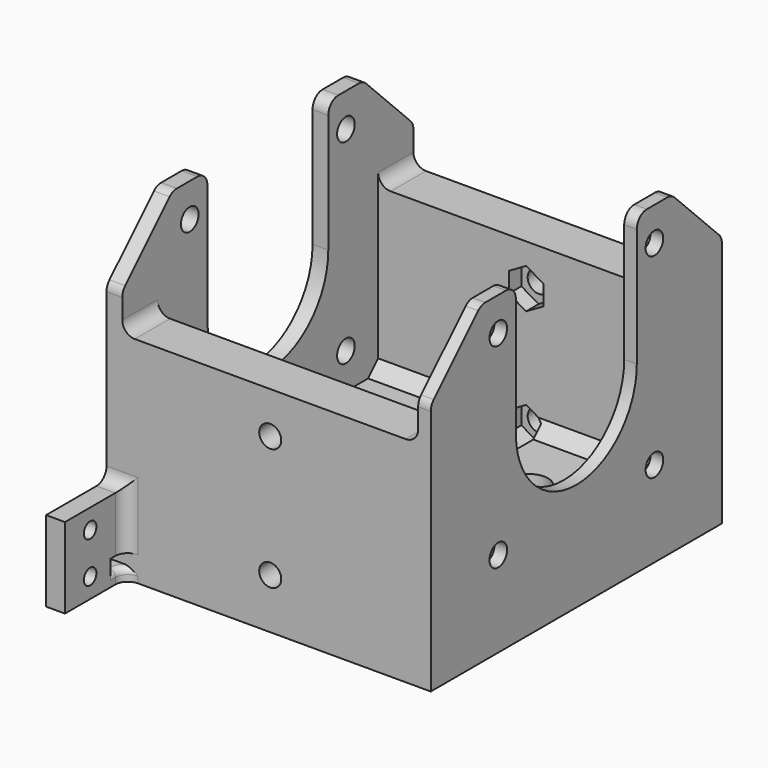
from build123d import *

# Parameters (mm, degrees)
F1_W         = 27
F1_H         = 43.8
F1_R         = 1.5
F1_H_2       = 7
F2_DEPTH     = 34
F3_R         = 1.75
F4_DEPTH     = 57.801
F5_W         = 43.8
F5_H         = 26
F6_DEPTH     = 27.001
F7_DEPTH     = 10
F8_DEPTH     = 10
F9_T4_DEPTH  = 26.8933659759
F9_S5_R      = 1.75
F9_T6_DEPTH  = 15
F9_T10_DEPTH = 26.8933659759
F9_S11_R     = 1.75
F9_T12_DEPTH = 15
F9_T16_DEPTH = 26.8933659759
F9_S17_R     = 1.75
F9_T18_DEPTH = 15
F9_T22_DEPTH = 26.8933659759
F9_S23_R     = 1.75
F9_T24_DEPTH = 15
F12_DEPTH    = 2.5
F14_DEPTH    = 2
F15_SIZE     = 10
F16_R        = 1.75
F17_DEPTH    = 51.5
F18_R        = 3
F19_DEPTH    = 4
F21_DEPTH    = 2.5
F22_DEPTH    = 47
F24_DEPTH    = 2.5
F25_R        = 1.25
F26_DEPTH    = 3
F27_R        = 2
F28_T1_DEPTH = 1
F28_T3_DEPTH = 3
F28_T8_ANGLE = 161.6484946187


# Not quite as in the source:
# - a fillet or chamfer that OpenCascade refuses, or shapes differently, is made with other operations: its cross-section is extruded or revolved along the edge and cut away or added


with BuildPart() as f2:
    # F1 (on Top) → F2 (new body)
    with BuildSketch(Plane.XY):
        Rectangle(F1_W, F1_H)
        with Locations((-10, -10)):
            Circle(F1_R, mode=Mode.SUBTRACT)
        with Locations((10, -10)):
            Circle(F1_R, mode=Mode.SUBTRACT)
        with Locations((-10, 10)):
            Circle(F1_R, mode=Mode.SUBTRACT)
        with Locations((10, 10)):
            Circle(F1_R, mode=Mode.SUBTRACT)
        with Locations((0, 25.4)):
            Rectangle(F1_W, F1_H_2)
        with Locations((0, -25.4)):
            Rectangle(F1_W, F1_H_2)
    extrude(amount=F2_DEPTH)

    # F3 (on face) → F4 (cut, through all)
    with BuildSketch(Plane(origin=(0, 28.9, 0), x_dir=(-1, 0, 0), z_dir=(0, 1, 0))):
        with Locations((0, 27.395)):
            Circle(F3_R)
        with Locations((0, 8)):
            Circle(F3_R)
    extrude(amount=-F4_DEPTH, mode=Mode.SUBTRACT)

    # F5 (on face) → F6 (cut, through all)
    with BuildSketch(Plane(origin=(-13.5, 0, 0), x_dir=(0, -1, 0), z_dir=(-1, 0, 0))):
        with Locations((0, 21)):
            Rectangle(F5_W, F5_H)
    extrude(amount=-F6_DEPTH, mode=Mode.SUBTRACT)

    # F7 (add): a face of the model
    f7_faces = [f2.faces().sort_by_distance(p)[0] for p in [
        (-13.5, 0, 0.6705848194),
    ]]
    extrude(f7_faces, amount=F7_DEPTH)

    # F8 (add): a face of the model
    f8_faces = [f2.faces().sort_by_distance(p)[0] for p in [
        (13.5, 0, 0.6705848194),
    ]]
    extrude(f8_faces, amount=F8_DEPTH)

    # F9: chamfer of 2 on 4 edges, made by hand


with BuildPart() as f9_tool2:
    # F9_s3 → F9_t4 (new body)
    with BuildSketch(Plane.YZ.offset(3.3933659759)):
        Polygon((-21.9, 10), (-19.9, 8), (-21.9, 8), align=None)
    extrude(amount=-F9_T4_DEPTH)

    # F9_s5 → F9_t6 (cut, symmetric)
    with BuildSketch(Plane.XZ.offset(20.9)):
        with Locations((0, 8)):
            Circle(F9_S5_R)
    extrude(amount=F9_T6_DEPTH, both=True, mode=Mode.SUBTRACT)


with BuildPart() as f2_1:
    add(f2.part)

    # F9_t1: union F9_tool2
    add(f9_tool2.part)


with BuildPart() as f9_tool8:
    # F9_s9 → F9_t10 (new body)
    with BuildSketch(Plane.YZ.offset(-23.5)):
        Polygon((21.9, 10), (19.9, 8), (21.9, 8), align=None)
    extrude(amount=F9_T10_DEPTH)

    # F9_s11 → F9_t12 (cut, symmetric)
    with BuildSketch(Plane.XZ.offset(-20.9)):
        with Locations((0, 8)):
            Circle(F9_S11_R)
    extrude(amount=F9_T12_DEPTH, both=True, mode=Mode.SUBTRACT)


with BuildPart() as f2_2:
    add(f2_1.part)

    # F9_t7: union F9_tool8
    add(f9_tool8.part)


with BuildPart() as f9_tool14:
    # F9_s15 → F9_t16 (new body)
    with BuildSketch(Plane.YZ.offset(-3.3933659759)):
        Polygon((21.9, 10), (19.9, 8), (21.9, 8), align=None)
    extrude(amount=F9_T16_DEPTH)

    # F9_s17 → F9_t18 (cut, symmetric)
    with BuildSketch(Plane.XZ.offset(-20.9)):
        with Locations((0, 8)):
            Circle(F9_S17_R)
    extrude(amount=F9_T18_DEPTH, both=True, mode=Mode.SUBTRACT)


with BuildPart() as f2_3:
    add(f2_2.part)

    # F9_t13: union F9_tool14
    add(f9_tool14.part)


with BuildPart() as f9_tool20:
    # F9_s21 → F9_t22 (new body)
    with BuildSketch(Plane.YZ.offset(23.5)):
        Polygon((-19.9, 8), (-21.9, 10), (-21.9, 8), align=None)
    extrude(amount=-F9_T22_DEPTH)

    # F9_s23 → F9_t24 (cut, symmetric)
    with BuildSketch(Plane.XZ.offset(20.9)):
        with Locations((0, 8)):
            Circle(F9_S23_R)
    extrude(amount=F9_T24_DEPTH, both=True, mode=Mode.SUBTRACT)


with BuildPart() as f2_4:
    add(f2_3.part)

    # F9_t19: union F9_tool20
    add(f9_tool20.part)

    # F11 (on face) → F12 (join)
    with BuildSketch(Plane(origin=(-23.5, 0, 0), x_dir=(0, -1, 0), z_dir=(-1, 0, 0))):
        Polygon((-28.9, 50), (-28.9, 34), (-28.9, 0), (28.9, 0), (28.9, 50), align=None)
    extrude(amount=F12_DEPTH)

    # F13 (on face) → F14 (join)
    with BuildSketch(Plane.YZ.offset(23.5)):
        Polygon((-28.9, 34), (-28.9, 28), (-28.9, 0), (28.9, 0), (28.9, 28), (28.9, 34), (28.9, 50), (-28.9, 50), align=None)
    extrude(amount=F14_DEPTH)

    # F15
    f15_edges = [f2_4.edges().sort_by_distance(p)[0] for p in [
        (-24.75, 28.9, 50),
        (-24.75, -28.9, 50),
        (24.5, -28.9, 50),
        (24.5, 28.9, 50),
    ]]
    chamfer(f15_edges, length=F15_SIZE)

    # F16 (on face) → F17 (cut, through all)
    with BuildSketch(Plane.YZ.offset(25.5)):
        with BuildLine():
            Line((-12, 50), (-12, 29.15))
            ThreePointArc((-12, 29.15), (0, 17.15), (12, 29.15))
            Line((12, 29.15), (12, 50))
            Line((12, 50), (-12, 50))
        make_face()
        with Locations((-15.5, 44.65)):
            Circle(F16_R)
        with Locations((15.5, 44.65)):
            Circle(F16_R)
        with Locations((15.5, 13.65)):
            Circle(F16_R)
        with Locations((-15.5, 13.65)):
            Circle(F16_R)
    extrude(amount=-F17_DEPTH, mode=Mode.SUBTRACT)

    # F18 (on face) → F19 (cut)
    with BuildSketch(Plane.XY.offset(8)):
        with Locations((10, -10)):
            Circle(F18_R)
        with Locations((10, 10)):
            Circle(F18_R)
        with Locations((-10, -10)):
            Circle(F18_R)
        with Locations((-10, 10)):
            Circle(F18_R)
    extrude(amount=-F19_DEPTH, mode=Mode.SUBTRACT)

    # F20 (on face) → F21 (cut)
    with BuildSketch(Plane.XZ.offset(-21.9)):
        Polygon((2.75, 25.8072867597), (2.75, 28.9827132403), (0, 30.5704264805), (-2.75, 28.9827132403), (-2.75, 25.8072867597), (0, 24.2195735195), align=None)
        Polygon((2.75, 6.3760742294), (2.75, 9.55150071), (0, 11.1392139502), (-2.75, 9.55150071), (-2.75, 6.3760742294), (0, 4.7883609892), align=None)
    extrude(amount=-F21_DEPTH, mode=Mode.SUBTRACT)

    # F20 (on face) → F22 (cut)
    with BuildSketch(Plane.XZ.offset(-21.9)):
        Polygon((2.75, 6.3760742294), (2.75, 9.55150071), (1.9731764425, 10), (-1.9731764425, 10), (-2.75, 9.55150071), (-2.75, 6.3760742294), (0, 4.7883609892), align=None)
    extrude(amount=F22_DEPTH, mode=Mode.SUBTRACT)

    # F23 (on face) → F24 (cut)
    with BuildSketch(Plane(origin=(0, -21.9, 0), x_dir=(-1, 0, 0), z_dir=(0, 1, 0))):
        Polygon((2.75, 25.8072867597), (2.75, 28.9827132403), (0, 30.5704264805), (-2.75, 28.9827132403), (-2.75, 25.8072867597), (0, 24.2195735195), align=None)
        Polygon((2.75, 6.4122867597), (2.75, 9.5877132403), (0, 11.1754264805), (-2.75, 9.5877132403), (-2.75, 6.4122867597), (0, 4.8245735195), align=None)
    extrude(amount=-F24_DEPTH, mode=Mode.SUBTRACT)

    # F25 (on face) → F26 (join)
    with BuildSketch(Plane(origin=(-26, 0, 0), x_dir=(0, -1, 0), z_dir=(-1, 0, 0))):
        Polygon((28.9, 2), (28.9, 0), (40.9, 0), (40.9, 12.8), (28.9, 12.8), (28.9, 4), (31.9, 4), (31.9, 2), align=None)
        with Locations((35.9, 3.15)):
            Circle(F25_R, mode=Mode.SUBTRACT)
        with Locations((35.9, 9.65)):
            Circle(F25_R, mode=Mode.SUBTRACT)
    extrude(amount=-F26_DEPTH)

    # F27
    f27_edges = [f2_4.edges().sort_by_distance(p)[0] for p in [
        (-24.5, -28.9, 12.8),
        (23.5, -25.4, 34),
        (-23.5, -25.4, 34),
        (-23.5, 25.4, 34),
        (23.5, 25.4, 34),
        (-23, -28.9, 8.4),
        (-23, -28.9, 1),
        (24.5, 28.9, 40),
        (-24.75, 28.9, 40),
        (-24.75, 18.9, 50),
        (-24.75, -12, 50),
        (-24.75, 12, 50),
        (-24.75, -18.9, 50),
        (24.5, -12, 50),
        (24.5, 12, 50),
        (24.5, -18.9, 50),
        (24.5, -28.9, 40),
        (-24.75, -28.9, 40),
        (24.5, 18.9, 50),
    ]]
    fillet(f27_edges, radius=F27_R)

    # F28: fillet of radius 1 on 3 edges, made by hand

    # F28_s2 → F28_t1 (cut)
    with BuildSketch(Plane.XZ.offset(30.9)):
        with BuildLine():
            ThreePointArc((-24, 2), (-23.2928932188, 1.7071067812), (-23, 1))
            Line((-23, 1), (-23, 2))
            Line((-23, 2), (-24, 2))
        make_face()
    extrude(amount=F28_T1_DEPTH, mode=Mode.SUBTRACT)

    # F28_s4 → F28_t3 (cut)
    with BuildSketch(Plane.XZ.offset(28.9)):
        with BuildLine():
            ThreePointArc((-26, 1), (-25.7071067812, 1.7071067812), (-25, 2))
            Line((-25, 2), (-26, 2))
            Line((-26, 2), (-26, 1))
        make_face()
    extrude(amount=F28_T3_DEPTH, mode=Mode.SUBTRACT)


with BuildPart() as f28_tool6:
    # F28_s7 → F28_t8 (revolve)
    with BuildSketch(Plane(origin=(7.1522739521, -21.561442082, 0), x_dir=(0, 0, 1), z_dir=(0.3148458041, -0.9491428342, 0))):
        with BuildLine():
            ThreePointArc((2, 26.6607348638), (1.7071067812, 27.367841645), (1, 27.6607348638))
            Line((1, 27.6607348638), (2, 27.6607348638))
            Line((2, 27.6607348638), (2, 26.6607348638))
        make_face()
    revolve(axis=Axis((-21, -30.9, 2), (0, 0, 1)), revolution_arc=F28_T8_ANGLE)

    split(bisect_by=Plane.XZ.offset(28.9), keep=Keep.TOP)


with BuildPart() as f2_5:
    add(f2_4.part)

    # F28_t5: cut F28_tool6
    add(f28_tool6.part, mode=Mode.SUBTRACT)


solid = f2_5.part
